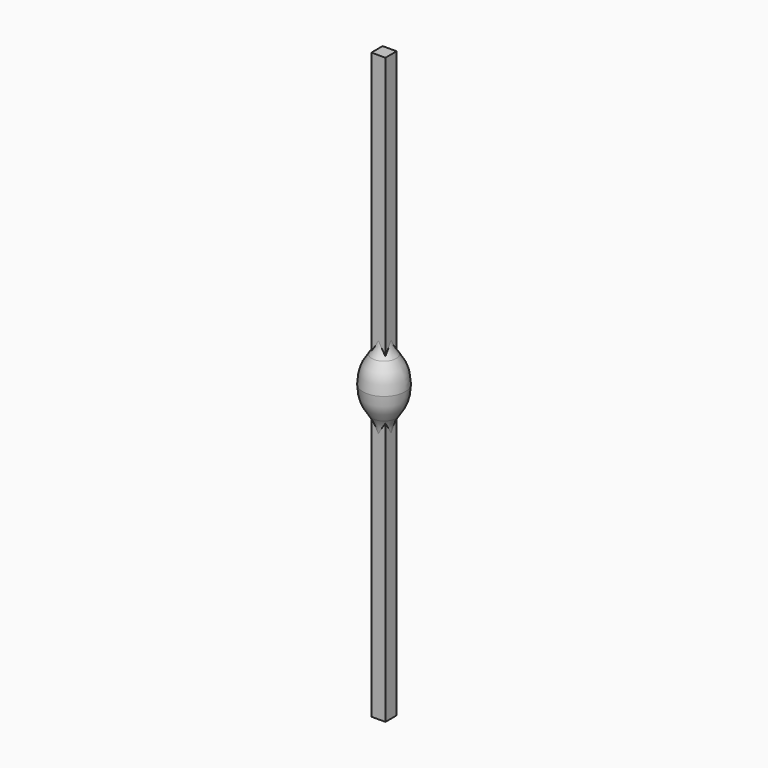
from build123d import *

# Parameters (mm, degrees)
F3_DEPTH      = 210
F3_DEPTH_BACK = 25
F5_DEPTH      = 210
F5_DEPTH_BACK = 25


with BuildPart() as f1:
    # F0 (on Front) → F1 (revolve)
    with BuildSketch(Plane.XZ):
        with BuildLine():
            Line((6, 40), (0, 40))
            Line((0, 40), (0, -40))
            Line((0, -40), (6, -40))
            Line((6, -40), (6, -35))
            ThreePointArc((6, -35), (7.121945325, -28.3955279025), (10.3619051686, -22.5320414644))
            ThreePointArc((10.3619051686, -22.5320414644), (16.1478700246, -11.9337677658), (17.9879737223, 0))
            ThreePointArc((17.9879737223, 0), (16.1478700246, 11.9337677658), (10.3619051686, 22.5320414644))
            ThreePointArc((10.3619051686, 22.5320414644), (7.121945325, 28.3955279025), (6, 35))
            Line((6, 35), (6, 40))
        make_face()
    revolve(axis=Axis((0, 0, 0), (0, 0, -1)))

    # F2 (on face) → F3 (join, two sides)
    with BuildSketch(Plane.XY.offset(40)) as f3_sk:
        with BuildLine():
            Line((6, 0), (6, 6))
            Line((6, 6), (0, 6))
            ThreePointArc((0, 6), (4.2426406871, 4.2426406871), (6, 0))
        make_face()
        with BuildLine():
            ThreePointArc((-6, 0), (-4.2426406871, 4.2426406871), (0, 6))
            Line((0, 6), (-6, 6))
            Line((-6, 6), (-6, 0))
        make_face()
        with BuildLine():
            ThreePointArc((0, -6), (-4.2426406871, -4.2426406871), (-6, 0))
            Line((-6, 0), (-6, -6))
            Line((-6, -6), (0, -6))
        make_face()
        with BuildLine():
            Line((6, -6), (6, 0))
            ThreePointArc((6, 0), (4.2426406871, -4.2426406871), (0, -6))
            Line((0, -6), (6, -6))
        make_face()
        with BuildLine():
            ThreePointArc((6, 0), (4.2426406871, 4.2426406871), (0, 6))
            ThreePointArc((0, 6), (-4.2426406871, 4.2426406871), (-6, 0))
            ThreePointArc((-6, 0), (-4.2426406871, -4.2426406871), (0, -6))
            ThreePointArc((0, -6), (4.2426406871, -4.2426406871), (6, 0))
        make_face()
    extrude(amount=F3_DEPTH)
    extrude(f3_sk.sketch, amount=-F3_DEPTH_BACK)

    # F4 (on face) → F5 (join, two sides)
    with BuildSketch(Plane(origin=(0, 0, -40), x_dir=(1, 0, 0), z_dir=(0, 0, -1))) as f5_sk:
        with BuildLine():
            Line((6, 0), (6, 6))
            Line((6, 6), (0, 6))
            ThreePointArc((0, 6), (4.2426406871, 4.2426406871), (6, 0))
        make_face()
        with BuildLine():
            ThreePointArc((-6, 0), (-4.2426406871, 4.2426406871), (0, 6))
            Line((0, 6), (-6, 6))
            Line((-6, 6), (-6, 0))
        make_face()
        with BuildLine():
            ThreePointArc((6, 0), (4.2426406871, 4.2426406871), (0, 6))
            ThreePointArc((0, 6), (-4.2426406871, 4.2426406871), (-6, 0))
            ThreePointArc((-6, 0), (-4.2426406871, -4.2426406871), (0, -6))
            ThreePointArc((0, -6), (4.2426406871, -4.2426406871), (6, 0))
        make_face()
        with BuildLine():
            Line((6, -6), (6, 0))
            ThreePointArc((6, 0), (4.2426406871, -4.2426406871), (0, -6))
            Line((0, -6), (6, -6))
        make_face()
        with BuildLine():
            ThreePointArc((0, -6), (-4.2426406871, -4.2426406871), (-6, 0))
            Line((-6, 0), (-6, -6))
            Line((-6, -6), (0, -6))
        make_face()
    extrude(amount=F5_DEPTH)
    extrude(f5_sk.sketch, amount=-F5_DEPTH_BACK)


solid = f1.part
